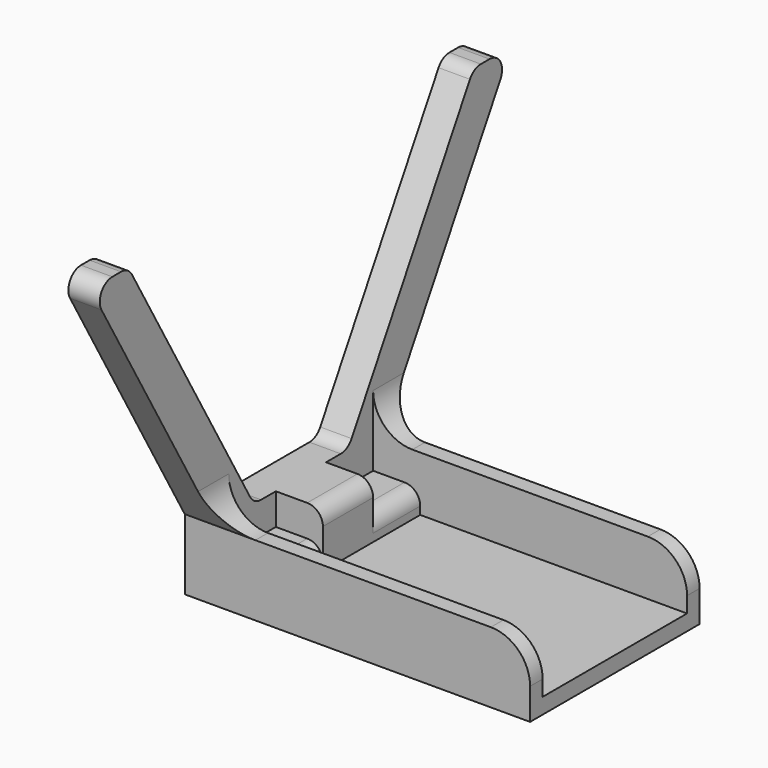
from build123d import *

# Parameters (mm, degrees)
F0_W      = 44
F0_H      = 27
F1_DEPTH  = 9
F2_W      = 34
F2_H      = 23
F3_DEPTH  = 7
F6_W      = 6
F6_H      = 7.5
F7_DEPTH  = 4
F5_W      = 6
F5_H      = 7.5
F10_DEPTH = 4
F12_DEPTH = 5
F14_R     = 2
F15_R     = 5


with BuildPart() as f1:
    # F0 (on Top) → F1 (new body)
    with BuildSketch(Plane.XY):
        with Locations((-1, 0)):
            Rectangle(F0_W, F0_H)
    extrude(amount=-F1_DEPTH)


with BuildPart() as f3:
    # F2 (on Top) → F3 (new body)
    with BuildSketch(Plane.XY):
        with Locations((4, 0)):
            Rectangle(F2_W, F2_H)
    extrude(amount=-F3_DEPTH)


with BuildPart() as f1_1:
    add(f1.part)

    # F4: cut F3
    add(f3.part, mode=Mode.SUBTRACT)


with BuildPart() as f7:
    # F6 (on Top) → F7 (new body)
    with BuildSketch(Plane.XY):
        with Locations((-16, -7.75)):
            Rectangle(F6_W, F6_H)
    extrude(amount=-F7_DEPTH)


with BuildPart() as f7b:
    # F5 (on Top) → F7, piece 2 (new body)
    with BuildSketch(Plane.XY):
        with Locations((-16, 7.75)):
            Rectangle(F5_W, F5_H)
    extrude(amount=-F7_DEPTH)


with BuildPart() as f1_2:
    add(f1_1.part)

    # F8: cut F7b, F7
    add(f7b.part, mode=Mode.SUBTRACT)
    add(f7.part, mode=Mode.SUBTRACT)

    # F9 (on face) → F10 (join)
    with BuildSketch(Plane(origin=(-23, 0, 0), x_dir=(0, -1, 0), z_dir=(-1, 0, 0))):
        Polygon((-13.5, 0), (13.5, 0), (33.5, 34.6410161514), (-33.5, 34.6410161514), align=None)
    extrude(amount=-F10_DEPTH)


with BuildPart() as f12:
    # F11 (on face) → F12 (new body)
    with BuildSketch(Plane(origin=(-23, 0, 0), x_dir=(0, -1, 0), z_dir=(-1, 0, 0))):
        Polygon((-7.5, 0), (7.5, 0), (27.5, 34.6410161514), (-27.5, 34.6410161514), align=None)
    extrude(amount=-F12_DEPTH)


with BuildPart() as f1_3:
    add(f1_2.part)

    # F13: cut F12
    add(f12.part, mode=Mode.SUBTRACT)

    # F14
    f14_edges = [f1_3.edges().sort_by_distance(p)[0] for p in [
        (-21, 33.5, 34.641016),
        (-21, 27.5, 34.641016),
        (-21, -27.5, 34.641016),
        (-21, -33.5, 34.641016),
        (-21, -7.5, 0),
        (-21, 7.5, 0),
        (-13, 0, 0),
        (-13, 7.75, -4),
        (-13, -7.75, -4),
    ]]
    fillet(f14_edges, radius=F14_R)

    # F15
    f15_edges = [f1_3.edges().sort_by_distance(p)[0] for p in [
        (-19, -12.5, 0),
        (-19, 12.5, 0),
        (21, 12.5, 0),
        (21, -12.5, 0),
    ]]
    fillet(f15_edges, radius=F15_R)


solid = f1_3.part
